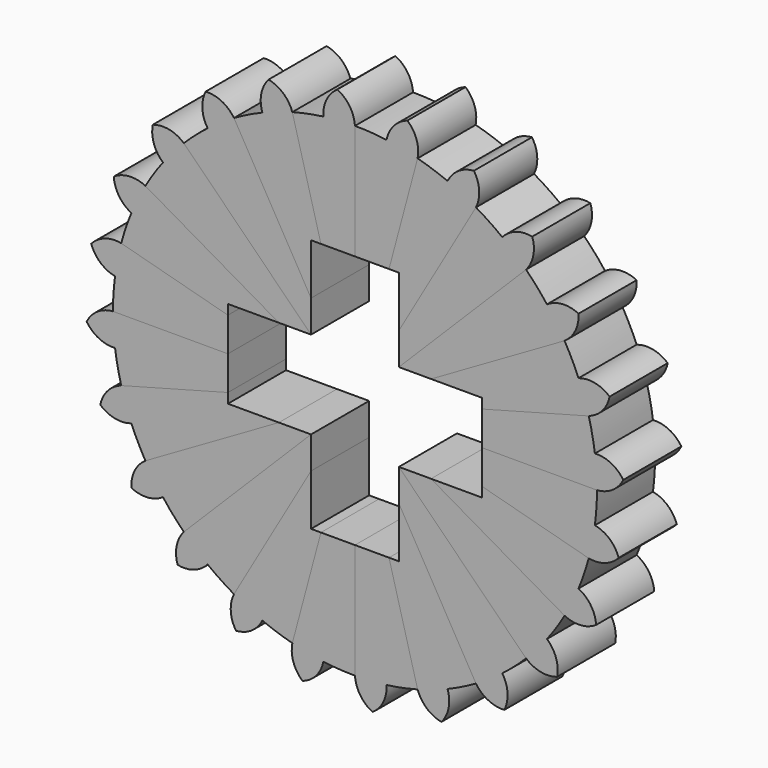
from build123d import *

# Parameters (mm, degrees)
F1_DEPTH = 7.62
F2_COUNT = 24
F2_ANGLE = 345
F3_W     = 8.7249
F3_H     = 9.2202
F3_W_2   = 9.2202
F3_H_2   = 8.7249
F4_DEPTH = 25.4


# Not quite as in the source:
# - a feature names something its author has since deleted; it is built from what else it names


with BuildPart() as f1:
    # F0 (on Front) → F1 (new body)
    with BuildSketch(Plane.XZ):
        with BuildLine():
            Line((24.5345159877, 6.5740037456), (0, 0))
            Line((0, 0), (25.4, 0))
            ThreePointArc((25.4, 0), (25.3456166503, 1.6612394824), (25.1826994789, 3.3153652824))
            ThreePointArc((25.1826994789, 3.3153652824), (24.9119461222, 4.9552941792), (24.5345159877, 6.5740037456))
        make_face()
        with BuildLine():
            ThreePointArc((25.1826994789, 3.3153652824), (25.3456166503, 1.6612394824), (25.4, 0))
            ThreePointArc((25.4, 0), (27.0285698916, 0.5528249856), (28.1625402968, 1.8458704127))
            ThreePointArc((28.1625402968, 1.8458704127), (26.8694948697, 2.9798408179), (25.1826994789, 3.3153652824))
        make_face()
    extrude(amount=F1_DEPTH)


with BuildPart() as f2_1:
    # F2: instance of F1
    add(f1.part.rotate(Axis((0, -3.81, 0), (0, 1, 0)), 1 * F2_ANGLE / (F2_COUNT - 1)))


with BuildPart() as f2_2:
    # F2: instance of F1
    add(f1.part.rotate(Axis((0, -3.81, 0), (0, 1, 0)), 2 * F2_ANGLE / (F2_COUNT - 1)))


with BuildPart() as f2_3:
    # F2: instance of F1
    add(f1.part.rotate(Axis((0, -3.81, 0), (0, 1, 0)), 3 * F2_ANGLE / (F2_COUNT - 1)))


with BuildPart() as f2_4:
    # F2: instance of F1
    add(f1.part.rotate(Axis((0, -3.81, 0), (0, 1, 0)), 4 * F2_ANGLE / (F2_COUNT - 1)))


with BuildPart() as f2_5:
    # F2: instance of F1
    add(f1.part.rotate(Axis((0, -3.81, 0), (0, 1, 0)), 5 * F2_ANGLE / (F2_COUNT - 1)))


with BuildPart() as f2_6:
    # F2: instance of F1
    add(f1.part.rotate(Axis((0, -3.81, 0), (0, 1, 0)), 6 * F2_ANGLE / (F2_COUNT - 1)))


with BuildPart() as f2_7:
    # F2: instance of F1
    add(f1.part.rotate(Axis((0, -3.81, 0), (0, 1, 0)), 7 * F2_ANGLE / (F2_COUNT - 1)))


with BuildPart() as f2_8:
    # F2: instance of F1
    add(f1.part.rotate(Axis((0, -3.81, 0), (0, 1, 0)), 8 * F2_ANGLE / (F2_COUNT - 1)))


with BuildPart() as f2_9:
    # F2: instance of F1
    add(f1.part.rotate(Axis((0, -3.81, 0), (0, 1, 0)), 9 * F2_ANGLE / (F2_COUNT - 1)))


with BuildPart() as f2_10:
    # F2: instance of F1
    add(f1.part.rotate(Axis((0, -3.81, 0), (0, 1, 0)), 10 * F2_ANGLE / (F2_COUNT - 1)))


with BuildPart() as f2_11:
    # F2: instance of F1
    add(f1.part.rotate(Axis((0, -3.81, 0), (0, 1, 0)), 11 * F2_ANGLE / (F2_COUNT - 1)))


with BuildPart() as f2_12:
    # F2: instance of F1
    add(f1.part.rotate(Axis((0, -3.81, 0), (0, 1, 0)), 12 * F2_ANGLE / (F2_COUNT - 1)))


with BuildPart() as f2_13:
    # F2: instance of F1
    add(f1.part.rotate(Axis((0, -3.81, 0), (0, 1, 0)), 13 * F2_ANGLE / (F2_COUNT - 1)))


with BuildPart() as f2_14:
    # F2: instance of F1
    add(f1.part.rotate(Axis((0, -3.81, 0), (0, 1, 0)), 14 * F2_ANGLE / (F2_COUNT - 1)))


with BuildPart() as f2_15:
    # F2: instance of F1
    add(f1.part.rotate(Axis((0, -3.81, 0), (0, 1, 0)), 15 * F2_ANGLE / (F2_COUNT - 1)))


with BuildPart() as f2_16:
    # F2: instance of F1
    add(f1.part.rotate(Axis((0, -3.81, 0), (0, 1, 0)), 16 * F2_ANGLE / (F2_COUNT - 1)))


with BuildPart() as f2_17:
    # F2: instance of F1
    add(f1.part.rotate(Axis((0, -3.81, 0), (0, 1, 0)), 17 * F2_ANGLE / (F2_COUNT - 1)))


with BuildPart() as f2_18:
    # F2: instance of F1
    add(f1.part.rotate(Axis((0, -3.81, 0), (0, 1, 0)), 18 * F2_ANGLE / (F2_COUNT - 1)))


with BuildPart() as f2_19:
    # F2: instance of F1
    add(f1.part.rotate(Axis((0, -3.81, 0), (0, 1, 0)), 19 * F2_ANGLE / (F2_COUNT - 1)))


with BuildPart() as f2_20:
    # F2: instance of F1
    add(f1.part.rotate(Axis((0, -3.81, 0), (0, 1, 0)), 20 * F2_ANGLE / (F2_COUNT - 1)))


with BuildPart() as f2_21:
    # F2: instance of F1
    add(f1.part.rotate(Axis((0, -3.81, 0), (0, 1, 0)), 21 * F2_ANGLE / (F2_COUNT - 1)))


with BuildPart() as f2_22:
    # F2: instance of F1
    add(f1.part.rotate(Axis((0, -3.81, 0), (0, 1, 0)), 22 * F2_ANGLE / (F2_COUNT - 1)))


with BuildPart() as f2_23:
    # F2: instance of F1
    add(f1.part.rotate(Axis((0, -3.81, 0), (0, 1, 0)), 23 * F2_ANGLE / (F2_COUNT - 1)))


with BuildPart() as f4_tool:
    # F3 (on Front) → F4 (new body)
    with BuildSketch(Plane.XZ):
        with Locations((8.97255, 0)):
            Rectangle(F3_W, F3_H)
        Rectangle(F3_W_2, F3_H)
        with Locations((0, 8.97255)):
            Rectangle(F3_W_2, F3_H_2)
        with Locations((-8.97255, 0)):
            Rectangle(F3_W, F3_H)
        with Locations((0, -8.97255)):
            Rectangle(F3_W_2, F3_H_2)
    extrude(amount=F4_DEPTH)


with BuildPart() as f1_1:
    add(f1.part)

    # F4: cut by f4_tool
    add(f4_tool.part, mode=Mode.SUBTRACT)


with BuildPart() as f2_1_1:
    add(f2_1.part)

    # F4: cut by f4_tool
    add(f4_tool.part, mode=Mode.SUBTRACT)


with BuildPart() as f2_2_1:
    add(f2_2.part)

    # F4: cut by f4_tool
    add(f4_tool.part, mode=Mode.SUBTRACT)


with BuildPart() as f2_3_1:
    add(f2_3.part)

    # F4: cut by f4_tool
    add(f4_tool.part, mode=Mode.SUBTRACT)


with BuildPart() as f2_4_1:
    add(f2_4.part)

    # F4: cut by f4_tool
    add(f4_tool.part, mode=Mode.SUBTRACT)


with BuildPart() as f2_5_1:
    add(f2_5.part)

    # F4: cut by f4_tool
    add(f4_tool.part, mode=Mode.SUBTRACT)


with BuildPart() as f2_6_1:
    add(f2_6.part)

    # F4: cut by f4_tool
    add(f4_tool.part, mode=Mode.SUBTRACT)


with BuildPart() as f2_7_1:
    add(f2_7.part)

    # F4: cut by f4_tool
    add(f4_tool.part, mode=Mode.SUBTRACT)


with BuildPart() as f2_8_1:
    add(f2_8.part)

    # F4: cut by f4_tool
    add(f4_tool.part, mode=Mode.SUBTRACT)


with BuildPart() as f2_9_1:
    add(f2_9.part)

    # F4: cut by f4_tool
    add(f4_tool.part, mode=Mode.SUBTRACT)


with BuildPart() as f2_10_1:
    add(f2_10.part)

    # F4: cut by f4_tool
    add(f4_tool.part, mode=Mode.SUBTRACT)


with BuildPart() as f2_11_1:
    add(f2_11.part)

    # F4: cut by f4_tool
    add(f4_tool.part, mode=Mode.SUBTRACT)


with BuildPart() as f2_12_1:
    add(f2_12.part)

    # F4: cut by f4_tool
    add(f4_tool.part, mode=Mode.SUBTRACT)


with BuildPart() as f2_13_1:
    add(f2_13.part)

    # F4: cut by f4_tool
    add(f4_tool.part, mode=Mode.SUBTRACT)


with BuildPart() as f2_14_1:
    add(f2_14.part)

    # F4: cut by f4_tool
    add(f4_tool.part, mode=Mode.SUBTRACT)


with BuildPart() as f2_15_1:
    add(f2_15.part)

    # F4: cut by f4_tool
    add(f4_tool.part, mode=Mode.SUBTRACT)


with BuildPart() as f2_16_1:
    add(f2_16.part)

    # F4: cut by f4_tool
    add(f4_tool.part, mode=Mode.SUBTRACT)


with BuildPart() as f2_17_1:
    add(f2_17.part)

    # F4: cut by f4_tool
    add(f4_tool.part, mode=Mode.SUBTRACT)


with BuildPart() as f2_18_1:
    add(f2_18.part)

    # F4: cut by f4_tool
    add(f4_tool.part, mode=Mode.SUBTRACT)


with BuildPart() as f2_19_1:
    add(f2_19.part)

    # F4: cut by f4_tool
    add(f4_tool.part, mode=Mode.SUBTRACT)


with BuildPart() as f2_20_1:
    add(f2_20.part)

    # F4: cut by f4_tool
    add(f4_tool.part, mode=Mode.SUBTRACT)


with BuildPart() as f2_21_1:
    add(f2_21.part)

    # F4: cut by f4_tool
    add(f4_tool.part, mode=Mode.SUBTRACT)


with BuildPart() as f2_22_1:
    add(f2_22.part)

    # F4: cut by f4_tool
    add(f4_tool.part, mode=Mode.SUBTRACT)


with BuildPart() as f2_23_1:
    add(f2_23.part)

    # F4: cut by f4_tool
    add(f4_tool.part, mode=Mode.SUBTRACT)


solid = Compound([f1_1.part, f2_1_1.part, f2_2_1.part, f2_3_1.part, f2_4_1.part, f2_5_1.part, f2_6_1.part, f2_7_1.part, f2_8_1.part, f2_9_1.part, f2_10_1.part, f2_11_1.part, f2_12_1.part, f2_13_1.part, f2_14_1.part, f2_15_1.part, f2_16_1.part, f2_17_1.part, f2_18_1.part, f2_19_1.part, f2_20_1.part, f2_21_1.part, f2_22_1.part, f2_23_1.part])
